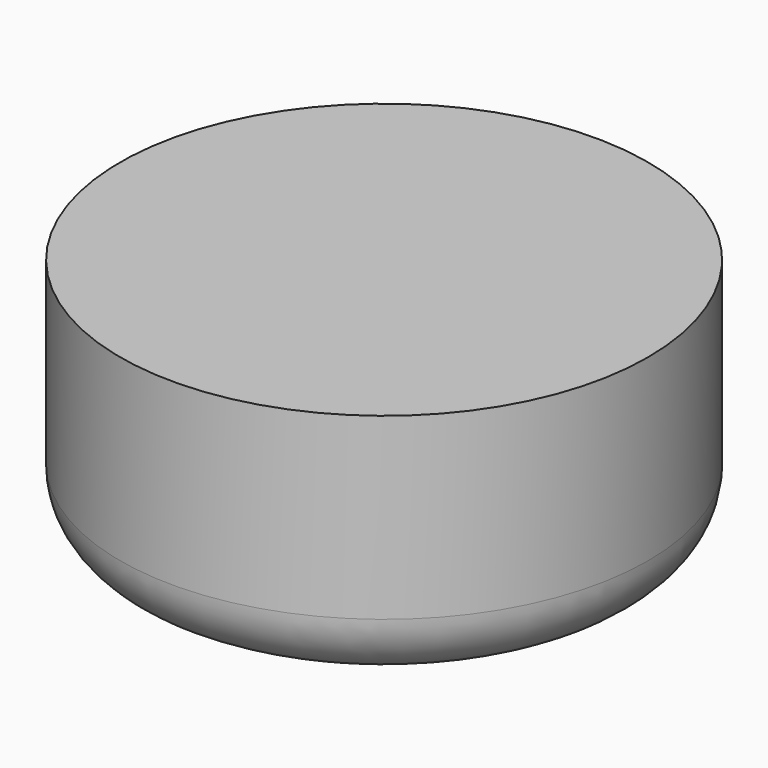
from build123d import *

# Parameters (mm, degrees)
F0_R         = 20.5792063899
F1_DEPTH     = 19.05
F5_R         = 5.08
F6_DEPTH     = 12.7
F7_TEXT_SIZE = 12.3629763645
F8_DEPTH     = 3.81


# Not quite as in the source:
# - the program builds the solid bodies; features that only make, move or delete a surface that nothing else refers to are left out
# - Text() gives the source's letters only with a copy of the font that has no kerning and outlines rounded to 1/6400 em; it was checked with that copy


with BuildPart() as f1:
    # F0 (on Top) → F1 (new body)
    with BuildSketch(Plane.XY):
        Circle(F0_R)
    extrude(amount=-F1_DEPTH)

    # F5
    f5_edges = [f1.edges().sort_by_distance(p)[0] for p in [
        (-20.579206, 0, -19.05),
    ]]
    fillet(f5_edges, radius=F5_R)

    # F6 (cut): a face of the model
    f6_faces = [f1.faces().sort_by_distance(p)[0] for p in [
        (0, 0, -19.05),
    ]]
    extrude(f6_faces, amount=-F6_DEPTH, mode=Mode.SUBTRACT)

    # F7 (on face) → F8 (join)
    with BuildSketch(Plane(origin=(0, 0, -6.35), x_dir=(1, 0, 0), z_dir=(0, 0, -1))):
        with Locations((-11.6933928803, -4.2183555197)):
            Text('KRB', F7_TEXT_SIZE, font='Open Sans', text_align=(TextAlign.LEFT, TextAlign.BOTTOM))
    extrude(amount=F8_DEPTH)


solid = f1.part
